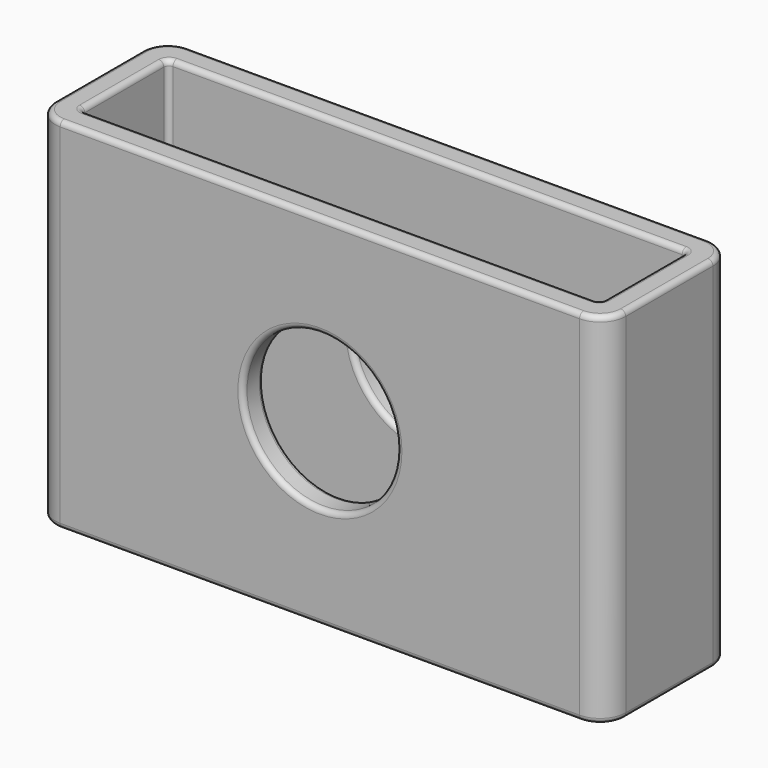
from build123d import *

# Parameters (mm, degrees)
F0_W     = 22.25
F0_H     = 6.25
F0_W_2   = 20.25
F0_H_2   = 4.25
F1_DEPTH = 14
F2_R     = 1
F3_R     = 0.2
F4_R     = 0.2
F5_R     = 3
F6_DEPTH = 6.251
F7_R     = 0.2


with BuildPart() as f1:
    # F0 (on Top) → F1 (new body)
    with BuildSketch(Plane.XY):
        Rectangle(F0_W, F0_H)
        Rectangle(F0_W_2, F0_H_2, mode=Mode.SUBTRACT)
    extrude(amount=F1_DEPTH)

    # F2
    f2_edges = [f1.edges().sort_by_distance(p)[0] for p in [
        (-11.125, -3.125, 7),
        (-11.125, 3.125, 7),
        (11.125, 3.125, 7),
        (11.125, -3.125, 7),
    ]]
    fillet(f2_edges, radius=F2_R)

    # F3
    f3_edges = [f1.edges().sort_by_distance(p)[0] for p in [
        (-10.125, 2.125, 7),
        (-10.125, -2.125, 7),
        (10.125, 2.125, 7),
        (10.125, -2.125, 7),
    ]]
    fillet(f3_edges, radius=F3_R)

    # F4
    f4_edges = [f1.edges().sort_by_distance(p)[0] for p in [
        (-10.832107, -2.832107, 14),
        (-10.832107, -2.832107, 0),
        (10.066421, -2.066421, 14),
        (10.066421, -2.066421, 0),
        (10.125, 0, 0),
        (10.066421, 2.066421, 0),
        (0, 2.125, 0),
        (0, -2.125, 0),
        (-10.066421, 2.066421, 0),
        (-10.066421, -2.066421, 0),
        (-10.125, 0, 0),
        (11.125, 0, 0),
        (10.832107, -2.832107, 0),
        (10.832107, 2.832107, 0),
        (0, -3.125, 0),
        (0, 3.125, 0),
        (-10.832107, 2.832107, 0),
        (-11.125, 0, 0),
        (10.125, 0, 14),
        (10.066421, 2.066421, 14),
        (0, 2.125, 14),
        (0, -2.125, 14),
        (-10.066421, 2.066421, 14),
        (-10.066421, -2.066421, 14),
        (-10.125, 0, 14),
        (11.125, 0, 14),
        (10.832107, -2.832107, 14),
        (10.832107, 2.832107, 14),
        (0, -3.125, 14),
        (0, 3.125, 14),
        (-10.832107, 2.832107, 14),
        (-11.125, 0, 14),
    ]]
    fillet(f4_edges, radius=F4_R)

    # F5 (on face) → F6 (cut, through all)
    with BuildSketch(Plane.XZ.offset(3.125)):
        with Locations((0, 7)):
            Circle(F5_R)
    extrude(amount=-F6_DEPTH, mode=Mode.SUBTRACT)

    # F7
    f7_edges = [f1.edges().sort_by_distance(p)[0] for p in [
        (-3, 3.125, 7),
        (-3, -3.125, 7),
        (-3, -2.125, 7),
        (-3, 2.125, 7),
    ]]
    fillet(f7_edges, radius=F7_R)


solid = f1.part
